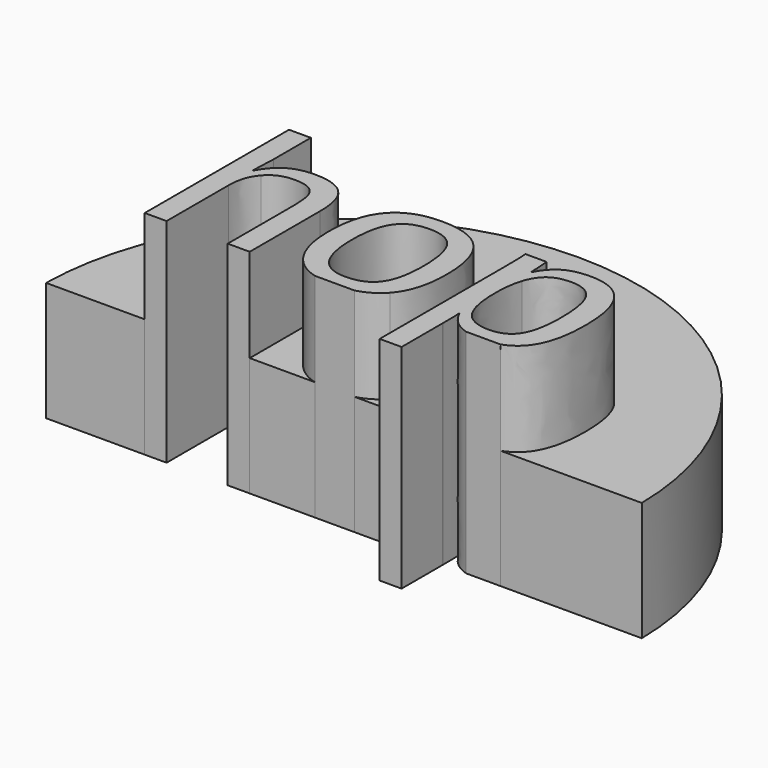
from build123d import *

# Parameters (mm, degrees)
F1_DEPTH = 25
F2_DEPTH = 14


with BuildPart() as f1:
    # F0 (on Top) → F1 (new body)
    with BuildSketch(Plane.XY):
        with BuildLine():
            Line((-12.7592669128, 21.1906875193), (-12.7592669128, 0))
            Line((-12.7592669128, 0), (-10.1915294428, 0))
            Line((-10.1915294428, 0), (-10.1915294428, 9.1104421978))
            add(Edge.make_bspline(
                [(-9.0995556789, 12.4914488309), (-10.1915294428, 11.2349936632), (-10.1915294428, 9.1104421978)],
                knots=[0, 0, 0, 1, 1, 1], degree=2))
            add(Edge.make_bspline(
                [(-6.1937175456, 13.7479039986), (-8.0075819149, 13.7479039986), (-9.0995556789, 12.4914488309)],
                knots=[0, 0, 0, 1, 1, 1], degree=2))
            add(Edge.make_bspline(
                [(-4.2930435464, 13.3778208401), (-4.9783827288, 13.7479039986), (-6.1937175456, 13.7479039986)],
                knots=[0, 0, 0, 1, 1, 1], degree=2))
            add(Edge.make_bspline(
                [(-3.3084395877, 12.215028694), (-3.607704364, 13.0077376816), (-4.2930435464, 13.3778208401)],
                knots=[0, 0, 0, 1, 1, 1], degree=2))
            add(Edge.make_bspline(
                [(-3.0091748114, 9.7957813802), (-3.0091748114, 11.4223197064), (-3.3084395877, 12.215028694)],
                knots=[0, 0, 0, 1, 1, 1], degree=2))
            Line((-3.0091748114, 9.7957813802), (-3.0091748114, 0))
            Line((-3.0091748114, 0), (-0.4231616299, 0))
            Line((-0.4231616299, 0), (-0.4231616299, 10.2937945194))
            add(Edge.make_bspline(
                [(-1.6156518072, 14.4857858516), (-0.4231616299, 13.2361840758), (-0.4231616299, 10.2937945194)],
                knots=[0, 0, 0, 1, 1, 1], degree=2))
            add(Edge.make_bspline(
                [(-5.32105232, 15.7353876275), (-2.8081419846, 15.7353876275), (-1.6156518072, 14.4857858516)],
                knots=[0, 0, 0, 1, 1, 1], degree=2))
            add(Edge.make_bspline(
                [(-8.2702952682, 15.0272038057), (-7.1075031221, 15.7353876275), (-5.32105232, 15.7353876275)],
                knots=[0, 0, 0, 1, 1, 1], degree=2))
            add(Edge.make_bspline(
                [(-10.260063361, 12.8067048548), (-9.4330874143, 14.3190199839), (-8.2702952682, 15.0272038057)],
                knots=[0, 0, 0, 1, 1, 1], degree=2))
            Line((-10.260063361, 12.8067048548), (-10.3057526399, 12.8067048548))
            add(Edge.make_bspline(
                [(-10.2417876495, 13.8781184433), (-10.2920458562, 12.9483416192), (-10.3057526399, 12.8067048548)],
                knots=[0, 0, 0, 1, 1, 1], degree=2))
            add(Edge.make_bspline(
                [(-10.1915294428, 15.675991565), (-10.1915294428, 14.8078952674), (-10.2417876495, 13.8781184433)],
                knots=[0, 0, 0, 1, 1, 1], degree=2))
            Line((-10.1915294428, 15.675991565), (-10.1915294428, 21.1906875193))
            Line((-10.1915294428, 21.1906875193), (-12.7592669128, 21.1906875193))
        make_face()
        with BuildLine():
            add(Edge.make_bspline(
                [(7.2449142086, 0), (5.51132105, 0.4831565087), (4.4290397814, 1.7773129463)],
                knots=[0.3733370206, 0.3733370206, 0.3733370206, 1, 1, 1], degree=2))
            Line((7.2449142086, 0), (11.8937666757, 0))
            add(Edge.make_bspline(
                [(14.7228343008, 1.6973567084), (13.6166302005, 0.4680838655), (11.8937666757, 0)],
                knots=[0, 0, 0, 0.6192188998, 0.6192188998, 0.6192188998], degree=2))
            add(Edge.make_bspline(
                [(16.5092851029, 7.739763833), (16.5092851029, 3.6825558733), (14.7228343008, 1.6973567084)],
                knots=[0, 0, 0, 1, 1, 1], degree=2))
            add(Edge.make_bspline(
                [(14.8370574978, 13.7867398856), (16.5092851029, 11.8380921437), (16.5092851029, 7.739763833)],
                knots=[0, 0, 0, 1, 1, 1], degree=2))
            add(Edge.make_bspline(
                [(9.6239107838, 15.7353876275), (13.1648298928, 15.7353876275), (14.8370574978, 13.7867398856)],
                knots=[0, 0, 0, 1, 1, 1], degree=2))
            add(Edge.make_bspline(
                [(2.7019850418, 7.739763833), (2.7019850418, 15.7353876275), (9.6239107838, 15.7353876275)],
                knots=[0, 0, 0, 1, 1, 1], degree=2))
            add(Edge.make_bspline(
                [(4.4290397814, 1.7773129463), (2.7019850418, 3.8424683492), (2.7019850418, 7.739763833)],
                knots=[0, 0, 0, 1, 1, 1], degree=2))
        make_face()
        with BuildLine():
            add(Edge.make_bspline(
                [(13.8090487243, 7.739763833), (13.8090487243, 10.9380133508), (12.8587117247, 12.3863634896)],
                knots=[0, 0, 0, 1, 1, 1], degree=2))
            add(Edge.make_bspline(
                [(12.8175913738, 3.0977331044), (13.8090487243, 4.5826346662), (13.8090487243, 7.739763833)],
                knots=[0, 0, 0, 1, 1, 1], degree=2))
            add(Edge.make_bspline(
                [(9.5096875868, 1.6128315425), (11.8261340232, 1.6128315425), (12.8175913738, 3.0977331044)],
                knots=[0, 0, 0, 1, 1, 1], degree=2))
            add(Edge.make_bspline(
                [(6.3913943069, 3.1479913111), (7.3851361214, 1.6128315425), (9.5096875868, 1.6128315425)],
                knots=[0, 0, 0, 1, 1, 1], degree=2))
            add(Edge.make_bspline(
                [(5.3976524925, 7.739763833), (5.3976524925, 4.6831510796), (6.3913943069, 3.1479913111)],
                knots=[0, 0, 0, 1, 1, 1], degree=2))
            add(Edge.make_bspline(
                [(6.4051010906, 12.3566654584), (5.3976524925, 10.8786172884), (5.3976524925, 7.739763833)],
                knots=[0, 0, 0, 1, 1, 1], degree=2))
            add(Edge.make_bspline(
                [(9.6696000627, 13.8347136284), (7.4125496887, 13.8347136284), (6.4051010906, 12.3566654584)],
                knots=[0, 0, 0, 1, 1, 1], degree=2))
            add(Edge.make_bspline(
                [(12.8587117247, 12.3863634896), (11.9083747251, 13.8347136284), (9.6696000627, 13.8347136284)],
                knots=[0, 0, 0, 1, 1, 1], degree=2))
        make_face(mode=Mode.SUBTRACT)
        with BuildLine():
            Line((25.0009693957, 0), (29.0291520059, 0))
            add(Edge.make_bspline(
                [(32.7700994369, 7.7945909676), (32.7700994369, 1.2374337453), (29.0291520059, 0)],
                knots=[0, 0, 0, 0.8112850274, 0.8112850274, 0.8112850274], degree=2))
            add(Edge.make_bspline(
                [(31.3560162572, 13.8073000611), (32.7700994369, 11.8929192783), (32.7700994369, 7.7945909676)],
                knots=[0, 0, 0, 1, 1, 1], degree=2))
            add(Edge.make_bspline(
                [(27.086353151, 15.7216808439), (29.9419330776, 15.7216808439), (31.3560162572, 13.8073000611)],
                knots=[0, 0, 0, 1, 1, 1], degree=2))
            add(Edge.make_bspline(
                [(24.1165500273, 15.056901837), (25.2450752143, 15.7216808439), (27.086353151, 15.7216808439)],
                knots=[0, 0, 0, 1, 1, 1], degree=2))
            add(Edge.make_bspline(
                [(22.3026856579, 12.9666173307), (22.9880248403, 14.39212283), (24.1165500273, 15.056901837)],
                knots=[0, 0, 0, 1, 1, 1], degree=2))
            Line((22.3026856579, 12.9666173307), (22.2478585233, 12.9666173307))
            add(Edge.make_bspline(
                [(22.2113071003, 13.964928073), (22.2478585233, 13.2361840758), (22.2478585233, 12.9666173307)],
                knots=[0, 0, 0, 1, 1, 1], degree=2))
            add(Edge.make_bspline(
                [(22.145057646, 15.0431950533), (22.1747556772, 14.6936720703), (22.2113071003, 13.964928073)],
                knots=[0, 0, 0, 1, 1, 1], degree=2))
            add(Edge.make_bspline(
                [(22.1016528311, 15.4475451709), (22.1153596148, 15.3927180363), (22.145057646, 15.0431950533)],
                knots=[0, 0, 0, 1, 1, 1], degree=2))
            Line((22.1016528311, 15.4475451709), (19.6207249909, 15.4475451709))
            add(Edge.make_bspline(
                [(19.7029656928, 12.294984932), (19.7029656928, 14.6799652867), (19.6207249909, 15.4475451709)],
                knots=[0, 0, 0, 1, 1, 1], degree=2))
            Line((19.7029656928, 12.294984932), (19.7029656928, 0))
            Line((19.7029656928, 0), (22.2752699909, 0))
            add(Edge.make_bspline(
                [(22.2158760282, 2.3986871383), (22.2749189421, 2.2851430731), (22.2752699909, 0)],
                knots=[0, 0, 0, 0.9940543441, 0.9940543441, 0.9940543441], degree=2))
            Line((22.2158760282, 2.3986871383), (22.2889788743, 2.3986871383))
            add(Edge.make_bspline(
                [(25.0009693957, 0), (23.1157221771, 0.5915307738), (22.2889788743, 2.3986871383)],
                knots=[0.3273268354, 0.3273268354, 0.3273268354, 1, 1, 1], degree=2))
        make_face()
        with BuildLine():
            add(Edge.make_bspline(
                [(30.0698630583, 7.739763833), (30.0698630583, 10.9654269181), (29.1994822967, 12.3498120665)],
                knots=[0, 0, 0, 1, 1, 1], degree=2))
            add(Edge.make_bspline(
                [(29.1926289048, 3.0200613304), (30.0698630583, 4.4272911182), (30.0698630583, 7.739763833)],
                knots=[0, 0, 0, 1, 1, 1], degree=2))
            add(Edge.make_bspline(
                [(26.4010139686, 1.6128315425), (28.3153947514, 1.6128315425), (29.1926289048, 3.0200613304)],
                knots=[0, 0, 0, 1, 1, 1], degree=2))
            add(Edge.make_bspline(
                [(23.2461692657, 3.0543282895), (24.2170664407, 1.6128315425), (26.4010139686, 1.6128315425)],
                knots=[0, 0, 0, 1, 1, 1], degree=2))
            add(Edge.make_bspline(
                [(22.2752720906, 7.5387310062), (22.2752720906, 4.4958250364), (23.2461692657, 3.0543282895)],
                knots=[0, 0, 0, 1, 1, 1], degree=2))
            add(Edge.make_bspline(
                [(22.7253114871, 11.086503507), (22.2752720906, 9.7226785341), (22.2752720906, 7.5387310062)],
                knots=[0, 0, 0, 1, 1, 1], degree=2))
            add(Edge.make_bspline(
                [(24.0388782533, 13.0922628475), (23.1753508835, 12.45032848), (22.7253114871, 11.086503507)],
                knots=[0, 0, 0, 1, 1, 1], degree=2))
            add(Edge.make_bspline(
                [(26.4284275359, 13.734197215), (24.9024056231, 13.734197215), (24.0388782533, 13.0922628475)],
                knots=[0, 0, 0, 1, 1, 1], degree=2))
            add(Edge.make_bspline(
                [(29.1994822967, 12.3498120665), (28.329101535, 13.734197215), (26.4284275359, 13.734197215)],
                knots=[0, 0, 0, 1, 1, 1], degree=2))
        make_face(mode=Mode.SUBTRACT)
        with BuildLine():
            add(Edge.make_bspline(
                [(22.2752699909, 0), (22.2752720906, -0.0136679392), (22.2752720906, -0.0274135673)],
                knots=[0.9940543441, 0.9940543441, 0.9940543441, 1, 1, 1], degree=2))
            Line((22.2752699909, 0), (19.7029656928, 0))
            Line((19.7029656928, 0), (19.7029656928, -6.067536228))
            Line((19.7029656928, -6.067536228), (22.2752720906, -6.067536228))
            Line((22.2752720906, -6.067536228), (22.2752720906, -0.0274135673))
        make_face()
    extrude(amount=F1_DEPTH)


with BuildPart() as f2:
    # F0 (on Top) → F2 (new body)
    with BuildSketch(Plane.XY):
        with BuildLine():
            ThreePointArc((45.649356842, 0), (10.649356842, 34.4880780529), (-24.350643158, 0))
            Line((-24.350643158, 0), (-12.7592669128, 0))
            Line((-12.7592669128, 0), (-12.7592669128, 21.1906875193))
            Line((-12.7592669128, 21.1906875193), (-10.1915294428, 21.1906875193))
            Line((-10.1915294428, 21.1906875193), (-10.1915294428, 15.675991565))
            add(Edge.make_bspline(
                [(-10.1915294428, 15.675991565), (-10.1915294428, 14.8078952674), (-10.2417876495, 13.8781184433)],
                knots=[0, 0, 0, 1, 1, 1], degree=2))
            add(Edge.make_bspline(
                [(-10.2417876495, 13.8781184433), (-10.2920458562, 12.9483416192), (-10.3057526399, 12.8067048548)],
                knots=[0, 0, 0, 1, 1, 1], degree=2))
            Line((-10.3057526399, 12.8067048548), (-10.260063361, 12.8067048548))
            add(Edge.make_bspline(
                [(-10.260063361, 12.8067048548), (-9.4330874143, 14.3190199839), (-8.2702952682, 15.0272038057)],
                knots=[0, 0, 0, 1, 1, 1], degree=2))
            add(Edge.make_bspline(
                [(-8.2702952682, 15.0272038057), (-7.1075031221, 15.7353876275), (-5.32105232, 15.7353876275)],
                knots=[0, 0, 0, 1, 1, 1], degree=2))
            add(Edge.make_bspline(
                [(-5.32105232, 15.7353876275), (-2.8081419846, 15.7353876275), (-1.6156518072, 14.4857858516)],
                knots=[0, 0, 0, 1, 1, 1], degree=2))
            add(Edge.make_bspline(
                [(-1.6156518072, 14.4857858516), (-0.4231616299, 13.2361840758), (-0.4231616299, 10.2937945194)],
                knots=[0, 0, 0, 1, 1, 1], degree=2))
            Line((-0.4231616299, 10.2937945194), (-0.4231616299, 0))
            Line((-0.4231616299, 0), (7.2449142086, 0))
            add(Edge.make_bspline(
                [(7.2449142086, 0), (5.51132105, 0.4831565087), (4.4290397814, 1.7773129463)],
                knots=[0.3733370206, 0.3733370206, 0.3733370206, 1, 1, 1], degree=2))
            add(Edge.make_bspline(
                [(4.4290397814, 1.7773129463), (2.7019850418, 3.8424683492), (2.7019850418, 7.739763833)],
                knots=[0, 0, 0, 1, 1, 1], degree=2))
            add(Edge.make_bspline(
                [(2.7019850418, 7.739763833), (2.7019850418, 15.7353876275), (9.6239107838, 15.7353876275)],
                knots=[0, 0, 0, 1, 1, 1], degree=2))
            add(Edge.make_bspline(
                [(9.6239107838, 15.7353876275), (13.1648298928, 15.7353876275), (14.8370574978, 13.7867398856)],
                knots=[0, 0, 0, 1, 1, 1], degree=2))
            add(Edge.make_bspline(
                [(14.8370574978, 13.7867398856), (16.5092851029, 11.8380921437), (16.5092851029, 7.739763833)],
                knots=[0, 0, 0, 1, 1, 1], degree=2))
            add(Edge.make_bspline(
                [(16.5092851029, 7.739763833), (16.5092851029, 3.6825558733), (14.7228343008, 1.6973567084)],
                knots=[0, 0, 0, 1, 1, 1], degree=2))
            add(Edge.make_bspline(
                [(14.7228343008, 1.6973567084), (13.6166302005, 0.4680838655), (11.8937666757, 0)],
                knots=[0, 0, 0, 0.6192188998, 0.6192188998, 0.6192188998], degree=2))
            Line((11.8937666757, 0), (19.7029656928, 0))
            Line((19.7029656928, 0), (19.7029656928, 12.294984932))
            add(Edge.make_bspline(
                [(19.7029656928, 12.294984932), (19.7029656928, 14.6799652867), (19.6207249909, 15.4475451709)],
                knots=[0, 0, 0, 1, 1, 1], degree=2))
            Line((19.6207249909, 15.4475451709), (22.1016528311, 15.4475451709))
            add(Edge.make_bspline(
                [(22.1016528311, 15.4475451709), (22.1153596148, 15.3927180363), (22.145057646, 15.0431950533)],
                knots=[0, 0, 0, 1, 1, 1], degree=2))
            add(Edge.make_bspline(
                [(22.145057646, 15.0431950533), (22.1747556772, 14.6936720703), (22.2113071003, 13.964928073)],
                knots=[0, 0, 0, 1, 1, 1], degree=2))
            add(Edge.make_bspline(
                [(22.2113071003, 13.964928073), (22.2478585233, 13.2361840758), (22.2478585233, 12.9666173307)],
                knots=[0, 0, 0, 1, 1, 1], degree=2))
            Line((22.2478585233, 12.9666173307), (22.3026856579, 12.9666173307))
            add(Edge.make_bspline(
                [(22.3026856579, 12.9666173307), (22.9880248403, 14.39212283), (24.1165500273, 15.056901837)],
                knots=[0, 0, 0, 1, 1, 1], degree=2))
            add(Edge.make_bspline(
                [(24.1165500273, 15.056901837), (25.2450752143, 15.7216808439), (27.086353151, 15.7216808439)],
                knots=[0, 0, 0, 1, 1, 1], degree=2))
            add(Edge.make_bspline(
                [(27.086353151, 15.7216808439), (29.9419330776, 15.7216808439), (31.3560162572, 13.8073000611)],
                knots=[0, 0, 0, 1, 1, 1], degree=2))
            add(Edge.make_bspline(
                [(31.3560162572, 13.8073000611), (32.7700994369, 11.8929192783), (32.7700994369, 7.7945909676)],
                knots=[0, 0, 0, 1, 1, 1], degree=2))
            add(Edge.make_bspline(
                [(32.7700994369, 7.7945909676), (32.7700994369, 1.2374337453), (29.0291520059, 0)],
                knots=[0, 0, 0, 0.8112850274, 0.8112850274, 0.8112850274], degree=2))
            Line((29.0291520059, 0), (45.649356842, 0))
        make_face()
    extrude(amount=F2_DEPTH)


solid = Compound([f1.part, f2.part])
